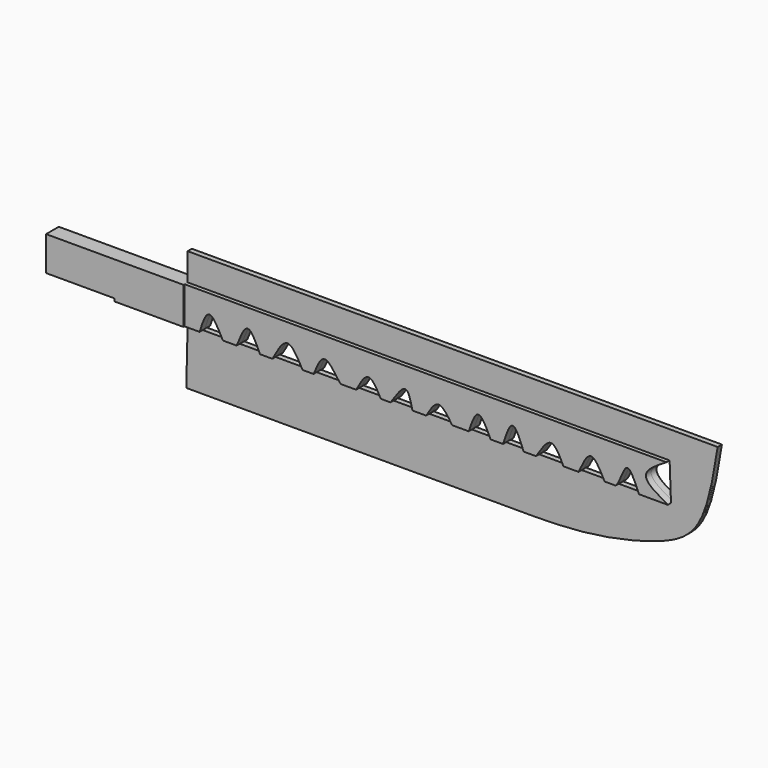
from build123d import *

# Parameters (mm, degrees)
F1_DEPTH = 1.27
F2_DEPTH = 3.81
F3_DEPTH = 3.175


# Not quite as in the source:
# - the program builds the solid bodies; features that only make, move or delete a surface that nothing else refers to are left out


with BuildPart() as f1:
    # F0 (on Front) → F1 (new body, symmetric)
    with BuildSketch(Plane.XZ):
        with BuildLine():
            Line((-210.2350903421, 55.0596148509), (-210.2350903421, 41.8989928542))
            Line((-210.2350903421, 41.8989928542), (20.7338259748, 41.8989928542))
            Line((20.7338259748, 41.8989928542), (21.3918573496, 24.1321539834))
            Line((21.3918573496, 24.1321539834), (7.5731984796, 24.1321539834))
            Line((7.5731984796, 24.1321539834), (-3.6133266435, 24.1321539834))
            add(Edge.make_bspline(
                [(-8.8775776416, 24.1321539834), (-6.9998897347, 23.4129011572), (-5.1222018278, 22.693648331), (-3.6133266435, 24.1321539834)],
                knots=[0, 0, 0, 0, 0.2589285415, 0.2589285415, 0.2589285415, 0.2589285415], degree=3))
            Line((-8.8775776416, 24.1321539834), (-21.3801710128, 24.1321539834))
            Line((-21.3801710128, 24.1321539834), (-28.6185133859, 24.1321539834))
            Line((-28.6185133859, 24.1321539834), (-41.7791353826, 24.1321539834))
            Line((-41.7791353826, 24.1321539834), (-47.7014150062, 24.1321539834))
            Line((-47.7014150062, 24.1321539834), (-57.5718773798, 24.1321539834))
            Line((-57.5718773798, 24.1321539834), (-63.4941570034, 24.1321539834))
            Line((-63.4941570034, 24.1321539834), (-74.0226589996, 24.1321539834))
            Line((-74.0226589996, 24.1321539834), (-81.9190354967, 24.1321539834))
            Line((-81.9190354967, 24.1321539834), (-94.4216164963, 24.1321539834))
            Line((-94.4216164963, 24.1321539834), (-101.0019316185, 24.1321539834))
            Line((-101.0019316185, 24.1321539834), (-111.5304336147, 24.1321539834))
            Line((-111.5304336147, 24.1321539834), (-116.1366559872, 24.1321539834))
            Line((-116.1366559872, 24.1321539834), (-127.9812152344, 24.1321539834))
            Line((-127.9812152344, 24.1321539834), (-133.903483861, 24.1321539834))
            add(Edge.make_bspline(
                [(-135.219563106, 24.1321539834), (-134.6550824726, 23.7299911861), (-134.2792831668, 23.9310725847), (-133.903483861, 24.1321539834)],
                knots=[0.8482904011, 0.8482904011, 0.8482904011, 0.8482904011, 1, 1, 1, 1], degree=3))
            Line((-135.219563106, 24.1321539834), (-148.3801796042, 24.1321539834))
            Line((-148.3801796042, 24.1321539834), (-153.6444306023, 24.1321539834))
            Line((-153.6444306023, 24.1321539834), (-168.1211043515, 24.1321539834))
            Line((-168.1211043515, 24.1321539834), (-174.0433949721, 24.1321539834))
            Line((-174.0433949721, 24.1321539834), (-185.2299145968, 24.1321539834))
            Line((-185.2299145968, 24.1321539834), (-191.8102228459, 24.1321539834))
            Line((-191.8102228459, 24.1321539834), (-202.9967644645, 24.1321539834))
            Line((-202.9967644645, 24.1321539834), (-210.2350903421, 24.1321539834))
            Line((-210.2350903421, 24.1321539834), (-210.8931299646, -2.8471227594))
            Line((-210.8931299646, -2.8471227594), (-54.9397518808, -2.8471227594))
            add(Edge.make_bspline(
                [(43.7649096579, 55.0596148509), (41.5344704617, 41.1814325972), (37.606662647, 16.7419263316), (16.1763288382, 4.9896597977), (-19.2697295543, -3.0062101287), (-43.0245937063, -2.9002640541), (-54.9397518808, -2.8471227594)],
                knots=[0, 0, 0, 0, 0.2688261018, 0.4734032944, 0.7358653369, 1, 1, 1, 1], degree=3))
            Line((43.7649096579, 55.0596148509), (-210.2350903421, 55.0596148509))
        make_face()
    extrude(amount=F1_DEPTH, both=True)


with BuildPart() as f2:
    # F0 (on Front) → F2 (new body, symmetric)
    with BuildSketch(Plane.XZ):
        Polygon((-259.5874352014, 41.8989928542), (-276.0382168211, 41.8989928542), (-276.0382168211, 25.4482167329), (-270.1159262005, 25.4482167329), align=None)
        Polygon((-250.3750014533, 41.8989928542), (-259.5874352014, 41.8989928542), (-270.1159262005, 25.4482167329), (-259.5874352014, 25.4482167329), align=None)
        Polygon((-243.1366535816, 41.8989928542), (-250.3750014533, 41.8989928542), (-259.5874352014, 25.4482167329), (-243.1366535816, 25.4482167329), align=None)
        Polygon((-226.6858719619, 41.8989928542), (-243.1366535816, 41.8989928542), (-243.1366535816, 25.4482167329), align=None)
        Polygon((-226.6858719619, 41.8989928542), (-243.1366535816, 25.4482167329), (-243.1366535816, 24.1321539834), (-233.266191208, 24.1321539834), (-218.7894954648, 41.8989928542), align=None)
        Polygon((-210.2350903421, 41.8989928542), (-218.7894954648, 41.8989928542), (-233.266191208, 24.1321539834), (-220.7635923383, 24.1321539834), (-210.2350903421, 33.0155734188), align=None)
        Polygon((-210.2350903421, 33.0155734188), (-220.7635923383, 24.1321539834), (-210.2350903421, 24.1321539834), align=None)
    extrude(amount=F2_DEPTH, both=True)


with BuildPart() as f3:
    # F0 (on Front) → F3 (new body, symmetric)
    with BuildSketch(Plane.XZ):
        with BuildLine():
            Line((20.7338259748, 41.8989928542), (-210.2350903421, 41.8989928542))
            Line((-210.2350903421, 41.8989928542), (-210.2350903421, 33.0155734188))
            Line((-210.2350903421, 33.0155734188), (-210.2350903421, 24.1321539834))
            Line((-210.2350903421, 24.1321539834), (-202.9967644645, 24.1321539834))
            add(Edge.make_bspline(
                [(-202.9967644645, 24.1321539834), (-201.5957848409, 28.5019031742), (-198.7222548422, 37.4646355189), (-194.1521756938, 28.6495004192), (-191.8102228459, 24.1321539834)],
                knots=[0, 0, 0, 0, 0.4875465453, 1, 1, 1, 1], degree=3))
            Line((-191.8102228459, 24.1321539834), (-185.2299145968, 24.1321539834))
            add(Edge.make_bspline(
                [(-185.2299145968, 24.1321539834), (-183.5214416822, 28.5493597006), (-180.0757441181, 37.4581078877), (-176.0653326357, 28.5987800772), (-174.0433949721, 24.1321539834)],
                knots=[0, 0, 0, 0, 0.4958278789, 1, 1, 1, 1], degree=3))
            Line((-174.0433949721, 24.1321539834), (-168.1211043515, 24.1321539834))
            add(Edge.make_bspline(
                [(-168.1211043515, 24.1321539834), (-165.7083305261, 28.5738628036), (-160.8827814128, 37.4572831365), (-156.0572146933, 28.5738645986), (-153.6444306023, 24.1321539834)],
                knots=[0, 0, 0, 0, 0.4999998484, 1, 1, 1, 1], degree=3))
            Line((-153.6444306023, 24.1321539834), (-148.3801796042, 24.1321539834))
            add(Edge.make_bspline(
                [(-148.3801796042, 24.1321539834), (-146.6101632269, 28.4123234005), (-142.9962239159, 37.1513795538), (-136.8299953213, 25.2795023356), (-135.219563106, 24.1321539834)],
                knots=[0, 0, 0, 0, 0.4154712555, 0.8482904011, 0.8482904011, 0.8482904011, 0.8482904011], degree=3))
            Line((-135.219563106, 24.1321539834), (-133.903483861, 24.1321539834))
            Line((-133.903483861, 24.1321539834), (-127.9812152344, 24.1321539834))
            add(Edge.make_bspline(
                [(-127.9812152344, 24.1321539834), (-126.0071220265, 27.75132517), (-122.0589356108, 34.9896675431), (-118.1107491951, 27.75132517), (-116.1366559872, 24.1321539834)],
                knots=[0, 0, 0, 0, 0.5, 1, 1, 1, 1], degree=3))
            Line((-116.1366559872, 24.1321539834), (-111.5304336147, 24.1321539834))
            add(Edge.make_bspline(
                [(-111.5304336147, 24.1321539834), (-108.8046270355, 28.2369832553), (-103.642943259, 36.0100331921), (-101.848674416, 27.9403570656), (-101.0019316185, 24.1321539834)],
                knots=[0, 0, 0, 0, 0.5280847679, 1, 1, 1, 1], degree=3))
            Line((-101.0019316185, 24.1321539834), (-94.4216164963, 24.1321539834))
            add(Edge.make_bspline(
                [(-94.4216164963, 24.1321539834), (-92.488331209, 27.3952792744), (-88.5729079881, 34.0039865465), (-84.1553655194, 27.4500227235), (-81.9190354967, 24.1321539834)],
                knots=[0, 0, 0, 0, 0.4937615114, 1, 1, 1, 1], degree=3))
            Line((-81.9190354967, 24.1321539834), (-74.0226589996, 24.1321539834))
            add(Edge.make_bspline(
                [(-74.0226589996, 24.1321539834), (-72.5787170502, 28.3613624742), (-69.6405343905, 36.967101131), (-65.5661989873, 28.4590196598), (-63.4941570034, 24.1321539834)],
                knots=[0, 0, 0, 0, 0.491440498, 1, 1, 1, 1], degree=3))
            Line((-63.4941570034, 24.1321539834), (-57.5718773798, 24.1321539834))
            add(Edge.make_bspline(
                [(-57.5718773798, 24.1321539834), (-56.084481964, 28.7157307739), (-53.0874293735, 37.9514864762), (-49.5056215462, 28.7613525636), (-47.7014150062, 24.1321539834)],
                knots=[0, 0, 0, 0, 0.496286058, 1, 1, 1, 1], degree=3))
            Line((-47.7014150062, 24.1321539834), (-41.7791353826, 24.1321539834))
            add(Edge.make_bspline(
                [(-41.7791353826, 24.1321539834), (-39.275468623, 28.135292461), (-34.3684870064, 35.9811157289), (-30.5088603888, 28.0275891282), (-28.6185133859, 24.1321539834)],
                knots=[0, 0, 0, 0, 0.5102254207, 1, 1, 1, 1], degree=3))
            Line((-28.6185133859, 24.1321539834), (-21.3801710128, 24.1321539834))
            add(Edge.make_bspline(
                [(-21.3801710128, 24.1321539834), (-19.4505524478, 28.3834837385), (-15.5556532425, 36.9647138246), (-11.1171492996, 28.4357047423), (-8.8775776416, 24.1321539834)],
                knots=[0, 0, 0, 0, 0.4954219514, 1, 1, 1, 1], degree=3))
            Line((-8.8775776416, 24.1321539834), (-3.6133266435, 24.1321539834))
            add(Edge.make_bspline(
                [(-3.6133266435, 24.1321539834), (-1.4711683739, 26.1744082476), (1.3487420826, 39.0591214669), (5.4874578129, 29.1340017152), (7.5731984796, 24.1321539834)],
                knots=[0.2589285415, 0.2589285415, 0.2589285415, 0.2589285415, 0.6265307939, 1, 1, 1, 1], degree=3))
            Line((7.5731984796, 24.1321539834), (21.3918573496, 24.1321539834))
            add(Edge.make_bspline(
                [(21.3918573496, 24.1321539834), (16.151488001, 27.0794656184), (5.7659846892, 32.9205261829), (15.7751403015, 38.9245229088), (20.7338259748, 41.8989928542)],
                knots=[0, 0, 0, 0, 0.5045850154, 1, 1, 1, 1], degree=3))
        make_face()
    extrude(amount=F3_DEPTH, both=True)


solid = Compound([f1.part, f2.part, f3.part])
